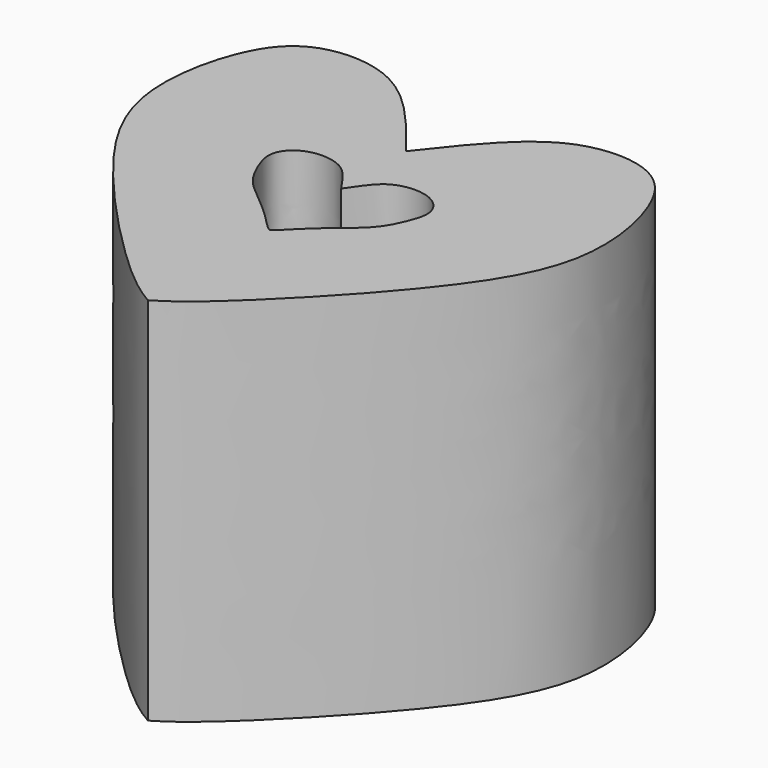
from build123d import *

# Parameters (mm, degrees)
F1_DEPTH = 33
F4_DEPTH = 76.9


# Not quite as in the source:
# - a feature names something its author has since deleted; it is built from what else it names


with BuildPart() as f1:
    # F0 (on Top) → F1 (new body)
    with BuildSketch(Plane.XY):
        with BuildLine():
            add(Edge.make_bspline(
                [(0, 10.2462833747), (2.8898270042, 13.9310457571), (7.0545812906, 19.2264572436), (15.3096506032, 19.2713715697), (18.952729902, 14.4439536567), (20.5921894779, 4.4447308225), (14.4997714791, -4.8290589443), (6.3713687355, -13.4563685464), (1.8976598298, -17.4473877844), (0, -18.5261424631)],
                knots=[0, 0, 0, 0, 0.161660753, 0.284836951, 0.395843898, 0.5421060645, 0.6997633553, 0.8663509734, 1, 1, 1, 1], degree=3))
            add(Edge.make_bspline(
                [(0, 10.2462833747), (-2.8898270042, 13.9310457571), (-7.0545812906, 19.2264572436), (-15.3096506032, 19.2713715697), (-18.952729902, 14.4439536567), (-20.5921894779, 4.4447308225), (-14.4997714791, -4.8290589443), (-6.3713687355, -13.4563685464), (-1.8976598298, -17.4473877844), (0, -18.5261424631)],
                knots=[0, 0, 0, 0, 0.161660753, 0.284836951, 0.395843898, 0.5421060645, 0.6997633553, 0.8663509734, 1, 1, 1, 1], degree=3))
        make_face()
    extrude(amount=F1_DEPTH)

    # F3 (on face) → F4 (cut)
    with BuildSketch(Plane.XY.offset(33)):
        with BuildLine():
            add(Edge.make_bspline(
                [(0, 3.0300645158), (0.6320519945, 3.8468260259), (1.7469002241, 6.0894075449), (5.5904577014, 6.3106402141), (7.4371838117, 4.2811169904), (6.6617686825, 1.9784920014), (5.6156573866, -0.1295622595), (3.2890882774, -1.9287685451), (1.4104347086, -3.5975135002), (0.4106112506, -4.7109916764), (0, -4.9717943184)],
                knots=[0, 0, 0, 0, 0.1417573032, 0.2836671205, 0.4010298291, 0.5158910582, 0.6354595782, 0.7678308655, 0.8938294053, 1, 1, 1, 1], degree=3))
            add(Edge.make_bspline(
                [(0, 3.0300645158), (-0.6320519945, 3.8468260259), (-1.7469002241, 6.0894075449), (-5.5904577014, 6.3106402141), (-7.4371838117, 4.2811169904), (-6.6617686825, 1.9784920014), (-5.6156573866, -0.1295622595), (-3.2890882774, -1.9287685451), (-1.4104347086, -3.5975135002), (-0.4106112506, -4.7109916764), (0, -4.9717943184)],
                knots=[0, 0, 0, 0, 0.1417573032, 0.2836671205, 0.4010298291, 0.5158910582, 0.6354595782, 0.7678308655, 0.8938294053, 1, 1, 1, 1], degree=3))
        make_face()
    extrude(amount=-F4_DEPTH, mode=Mode.SUBTRACT)


solid = f1.part
